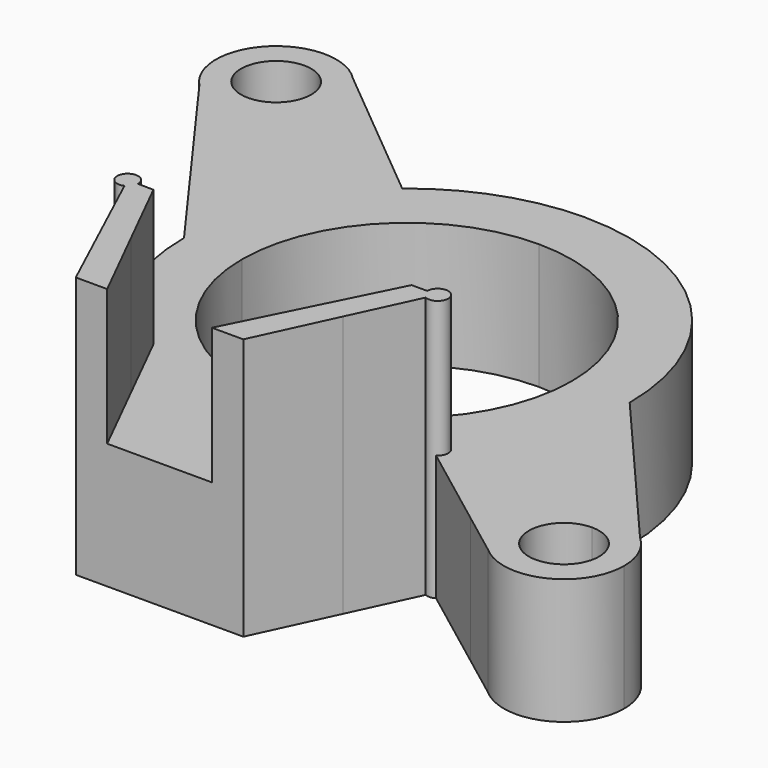
from build123d import *

# Parameters (mm, degrees)
F1_DEPTH = 12
F2_DEPTH = 25


with BuildPart() as f1:
    # F0 (on Top) → F1 (new body)
    with BuildSketch(Plane.XY):
        with BuildLine():
            ThreePointArc((-53.4150354704, 41.5196209399), (-52.7133447938, 40.4447331982), (-52.4674114412, 39.1848640586))
            Line((-52.4674114412, 39.1848640586), (-50.0674114412, 39.1848640586))
            ThreePointArc((-50.0674114412, 39.1848640586), (-50.4895358525, 41.3473260146), (-51.6939302973, 43.1922825863))
            Line((-51.6939302973, 43.1922825863), (-53.4150354704, 41.5196209399))
        make_face()
        with BuildLine():
            Line((-50.0674114412, 39.1848640586), (-52.4674114412, 39.1848640586))
            ThreePointArc((-52.4674114412, 39.1848640586), (-53.4486037242, 36.8160563416), (-55.8174114412, 35.8348640586))
            Line((-55.8174114412, 35.8348640586), (-55.8174114412, 33.4348640586))
            ThreePointArc((-55.8174114412, 33.4348640586), (-51.7515474493, 35.1190000668), (-50.0674114412, 39.1848640586))
        make_face()
        with BuildLine():
            ThreePointArc((-51.6939302973, 43.1922825863), (-50.4895358525, 41.3473260146), (-50.0674114412, 39.1848640586))
            Line((-50.0674114412, 39.1848640586), (-46.8600699283, 39.1848640586))
            Line((-46.8600699283, 39.1848640586), (-51.6939302973, 43.1922825863))
        make_face()
        with BuildLine():
            Line((-46.8600699283, 39.1848640586), (-50.0674114412, 39.1848640586))
            ThreePointArc((-50.0674114412, 39.1848640586), (-51.7515474493, 35.1190000668), (-55.8174114412, 33.4348640586))
            Line((-55.8174114412, 33.4348640586), (-55.8174114412, 29.501699648))
            Line((-55.8174114412, 29.501699648), (-45.4160998232, 15.1848640586))
            ThreePointArc((-45.4160998232, 15.1848640586), (-43.3893572478, 24.2490610317), (-37.6951490668, 31.5868635246))
            Line((-37.6951490668, 31.5868635246), (-46.8600699283, 39.1848640586))
        make_face()
        with BuildLine():
            Line((-55.8174114412, 33.4348640586), (-55.8174114412, 35.8348640586))
            ThreePointArc((-55.8174114412, 35.8348640586), (-57.1214560047, 36.099095471), (-58.219787412, 36.8501071773))
            Line((-58.219787412, 36.8501071773), (-59.9408925851, 35.177445531))
            ThreePointArc((-59.9408925851, 35.177445531), (-58.0556968861, 33.8883955874), (-55.8174114412, 33.4348640586))
        make_face()
        with BuildLine():
            ThreePointArc((-58.219787412, 36.8501071773), (-58.1521683225, 41.5872400294), (-53.4150354704, 41.5196209399))
            Line((-53.4150354704, 41.5196209399), (-51.6939302973, 43.1922825863))
            ThreePointArc((-51.6939302973, 43.1922825863), (-59.8248299688, 43.3083452025), (-59.9408925851, 35.177445531))
            Line((-59.9408925851, 35.177445531), (-58.219787412, 36.8501071773))
        make_face()
        with BuildLine():
            Line((-55.8174114412, 29.501699648), (-55.8174114412, 33.4348640586))
            ThreePointArc((-55.8174114412, 33.4348640586), (-58.0556968861, 33.8883955874), (-59.9408925851, 35.177445531))
            Line((-59.9408925851, 35.177445531), (-55.8174114412, 29.501699648))
        make_face()
        with BuildLine():
            ThreePointArc((-24.1338330771, 36.4671308048), (-31.3401896478, 35.2099309207), (-37.6951490668, 31.5868635246))
            ThreePointArc((-37.6951490668, 31.5868635246), (-43.3893572478, 24.2490610317), (-45.4160998232, 15.1848640586))
            Line((-45.4160998232, 15.1848640586), (-42.6338443592, 15.1848640586))
            Line((-42.6338443592, 15.1848640586), (-39.8838330771, 15.1848640586))
            ThreePointArc((-39.8838330771, 15.1848640586), (-35.2707648808, 26.3217958623), (-24.1338330771, 30.9348640586))
            Line((-24.1338330771, 30.9348640586), (-24.1338330771, 36.4671308048))
        make_face()
        with BuildLine():
            ThreePointArc((-2.8515663309, 15.1848640586), (-9.0849979418, 30.2336991939), (-24.1338330771, 36.4671308048))
            Line((-24.1338330771, 36.4671308048), (-24.1338330771, 30.9348640586))
            ThreePointArc((-24.1338330771, 30.9348640586), (-12.9969012734, 26.3217958623), (-8.3838330771, 15.1848640586))
            Line((-8.3838330771, 15.1848640586), (-5.6338443592, 15.1848640586))
            Line((-5.6338443592, 15.1848640586), (-2.8515663309, 15.1848640586))
        make_face()
        with BuildLine():
            Line((-42.6338443592, 15.1848640586), (-45.4160998232, 15.1848640586))
            ThreePointArc((-45.4160998232, 15.1848640586), (-43.9768109648, 7.4912884008), (-39.8536184288, 0.8383234878))
            ThreePointArc((-39.8536184288, 0.8383234878), (-38.7294279835, 1.3640933992), (-37.9593089049, 0.3908746355))
            ThreePointArc((-37.9593089049, 0.3908746355), (-37.9593613235, 0.3806357667), (-37.9595185738, 0.3703979712))
            Line((-37.9595185738, 0.3703979712), (-36.4598330771, 0.3396829748))
            Line((-36.4598330771, 0.3396829748), (-42.6338443592, 15.1848640586))
        make_face()
        with BuildLine():
            Line((7.549745287, 3.085096959), (-2.8515663309, 15.1848640586))
            Line((-2.8515663309, 15.1848640586), (-5.6338443592, 15.1848640586))
            Line((-5.6338443592, 15.1848640586), (-11.8078330771, 0.3396829748))
            Line((-11.8078330771, 0.3396829748), (-10.3078330771, 0.3396829748))
            ThreePointArc((-10.3078330771, 0.3396829748), (-9.3078330771, 1.3396829748), (-8.3078330771, 0.3396829748))
            ThreePointArc((-8.3078330771, 0.3396829748), (-8.4354300981, -0.1491043433), (-8.7856591617, -0.5131560499))
            Line((-8.7856591617, -0.5131560499), (-0.4328217774, -6.8151040581))
            Line((-0.4328217774, -6.8151040581), (1.9170580195, -6.8151040581))
            ThreePointArc((1.9170580195, -6.8151040581), (3.0940181915, -2.0251192122), (7.549745287, 0.0904625331))
            Line((7.549745287, 0.0904625331), (7.549745287, 3.085096959))
        make_face()
        with BuildLine():
            Line((-39.8838330771, 15.1848640586), (-42.6338443592, 15.1848640586))
            Line((-42.6338443592, 15.1848640586), (-36.4598330771, 0.3396829748))
            Line((-36.4598330771, 0.3396829748), (-29.3953061207, 0.3396829748))
            ThreePointArc((-29.3953061207, 0.3396829748), (-36.9971666349, 6.0965666504), (-39.8838330771, 15.1848640586))
        make_face()
        with BuildLine():
            ThreePointArc((-37.9593089049, 0.3908746355), (-38.7294279835, 1.3640933992), (-39.8536184288, 0.8383234878))
            ThreePointArc((-39.8536184288, 0.8383234878), (-39.649771274, 0.6181025887), (-39.4428392954, 0.4007778014))
            Line((-39.4428392954, 0.4007778014), (-38.9593089049, 0.3908746355))
            Line((-38.9593089049, 0.3908746355), (-37.9595185738, 0.3703979712))
            ThreePointArc((-37.9595185738, 0.3703979712), (-37.9593613235, 0.3806357667), (-37.9593089049, 0.3908746355))
        make_face()
        with BuildLine():
            ThreePointArc((-39.4428392954, 0.4007778014), (-39.649771274, 0.6181025887), (-39.8536184288, 0.8383234878))
            ThreePointArc((-39.8536184288, 0.8383234878), (-39.6769215407, -0.3055678279), (-38.5388324508, -0.5164288151))
            Line((-38.5388324508, -0.5164288151), (-38.5671831653, -0.4552536867))
            ThreePointArc((-38.5671831653, -0.4552536867), (-39.0111694362, -0.0335373263), (-39.4428392954, 0.4007778014))
        make_face()
        with BuildLine():
            Line((-5.6338443592, 15.1848640586), (-8.3838330771, 15.1848640586))
            ThreePointArc((-8.3838330771, 15.1848640586), (-11.2704995193, 6.0965666504), (-18.8723600334, 0.3396829748))
            Line((-18.8723600334, 0.3396829748), (-11.8078330771, 0.3396829748))
            Line((-11.8078330771, 0.3396829748), (-5.6338443592, 15.1848640586))
        make_face()
        with BuildLine():
            Line((11.3814063915, -1.3722454101), (7.549745287, 3.085096959))
            Line((7.549745287, 3.085096959), (7.549745287, 0.0904625331))
            ThreePointArc((7.549745287, 0.0904625331), (9.6004245249, -0.2876463043), (11.3814063915, -1.3722454101))
        make_face()
        with BuildLine():
            Line((-29.3953061207, 0.3396829748), (-36.4598330771, 0.3396829748))
            Line((-36.4598330771, 0.3396829748), (-32.8884867815, -6.8151040581))
            Line((-32.8884867815, -6.8151040581), (-24.1338330771, -6.8151040581))
            Line((-24.1338330771, -6.8151040581), (-24.1338330771, -0.5651359414))
            ThreePointArc((-24.1338330771, -0.5651359414), (-26.8031867376, -0.3372830556), (-29.3953061207, 0.3396829748))
        make_face()
        with BuildLine():
            Line((-32.8884867815, -6.8151040581), (-36.4598330771, 0.3396829748))
            Line((-36.4598330771, 0.3396829748), (-37.9595185738, 0.3703979712))
            ThreePointArc((-37.9595185738, 0.3703979712), (-38.1221082882, -0.1560212663), (-38.5388324508, -0.5164288151))
            Line((-38.5388324508, -0.5164288151), (-35.6198039494, -6.8151040581))
            Line((-35.6198039494, -6.8151040581), (-32.8884867815, -6.8151040581))
        make_face()
        with BuildLine():
            Line((-38.9593089049, 0.3908746355), (-39.4428392954, 0.4007778014))
            ThreePointArc((-39.4428392954, 0.4007778014), (-39.0111694362, -0.0335373263), (-38.5671831653, -0.4552536867))
            Line((-38.5671831653, -0.4552536867), (-38.9593089049, 0.3908746355))
        make_face()
        with BuildLine():
            Line((-38.5671831653, -0.4552536867), (-38.5388324508, -0.5164288151))
            ThreePointArc((-38.5388324508, -0.5164288151), (-38.1221082882, -0.1560212663), (-37.9595185738, 0.3703979712))
            Line((-37.9595185738, 0.3703979712), (-38.9593089049, 0.3908746355))
            Line((-38.9593089049, 0.3908746355), (-38.5671831653, -0.4552536867))
        make_face()
        with BuildLine():
            Line((-11.8078330771, 0.3396829748), (-18.8723600334, 0.3396829748))
            ThreePointArc((-18.8723600334, 0.3396829748), (-21.4644794165, -0.3372830556), (-24.1338330771, -0.5651359414))
            Line((-24.1338330771, -0.5651359414), (-24.1338330771, -6.8151040581))
            Line((-24.1338330771, -6.8151040581), (-15.3791793726, -6.8151040581))
            Line((-15.3791793726, -6.8151040581), (-11.8078330771, 0.3396829748))
        make_face()
        with BuildLine():
            Line((-10.3078330771, 0.3396829748), (-11.8078330771, 0.3396829748))
            Line((-11.8078330771, 0.3396829748), (-15.3791793726, -6.8151040581))
            Line((-15.3791793726, -6.8151040581), (-12.6354347442, -6.8151040581))
            Line((-12.6354347442, -6.8151040581), (-9.7295423368, -0.5670481321))
            ThreePointArc((-9.7295423368, -0.5670481321), (-10.1509550314, -0.1980394165), (-10.3078330771, 0.3396829748))
        make_face()
        with BuildLine():
            ThreePointArc((11.3814063915, -1.3722454101), (9.6004245249, -0.2876463043), (7.549745287, 0.0904625331))
            Line((7.549745287, 0.0904625331), (7.549745287, -2.3095374669))
            ThreePointArc((7.549745287, -2.3095374669), (8.744488843, -2.5298269634), (9.7821043653, -3.1617238338))
            Line((9.7821043653, -3.1617238338), (11.3814063915, -1.3722454101))
        make_face()
        with BuildLine():
            Line((7.549745287, -2.3095374669), (7.549745287, 0.0904625331))
            ThreePointArc((7.549745287, 0.0904625331), (3.0940181915, -2.0251192122), (1.9170580195, -6.8151040581))
            ThreePointArc((1.9170580195, -6.8151040581), (2.5652294004, -8.526086154), (3.7180841826, -9.9468295237))
            Line((3.7180841826, -9.9468295237), (5.3173862088, -8.1573511))
            ThreePointArc((5.3173862088, -8.1573511), (4.4200347836, -4.4647939109), (7.549745287, -2.3095374669))
        make_face()
        with BuildLine():
            ThreePointArc((13.299745287, -5.6595374669), (12.7982951511, -3.3110859931), (11.3814063915, -1.3722454101))
            Line((11.3814063915, -1.3722454101), (9.7821043653, -3.1617238338))
            ThreePointArc((9.7821043653, -3.1617238338), (10.6075960774, -4.291309217), (10.899745287, -5.6595374669))
            ThreePointArc((10.899745287, -5.6595374669), (8.917973537, -8.7173882573), (5.3173862088, -8.1573511))
            Line((5.3173862088, -8.1573511), (3.7180841826, -9.9468295237))
            ThreePointArc((3.7180841826, -9.9468295237), (9.8981967608, -10.9080873309), (13.299745287, -5.6595374669))
        make_face()
        Polygon((-24.1338330771, -6.8151040581), (-32.8884867815, -6.8151040581), (-29.1338330771, -14.3371266833), (-24.1338330771, -14.3371266833), (-24.1338330771, -7.8529477167), align=None)
        Polygon((-29.1338330771, -14.3371266833), (-32.8884867815, -6.8151040581), (-35.6198039494, -6.8151040581), (-32.1338330771, -14.3371266833), align=None)
        Polygon((-12.6354347442, -6.8151040581), (-15.3791793726, -6.8151040581), (-19.1338330771, -14.3371266833), (-16.1338330771, -14.3371266833), align=None)
        Polygon((-19.1338330771, -14.3371266833), (-15.3791793726, -6.8151040581), (-24.1338330771, -6.8151040581), (-24.1338330771, -7.8529477167), (-24.1338330771, -14.3371266833), align=None)
        with BuildLine():
            ThreePointArc((-8.3078330771, 0.3396829748), (-9.3078330771, 1.3396829748), (-10.3078330771, 0.3396829748))
            Line((-10.3078330771, 0.3396829748), (-9.3078330771, 0.3396829748))
            Line((-9.3078330771, 0.3396829748), (-9.4658153661, 0))
            Line((-9.4658153661, 0), (-8.7856591617, -0.5131560499))
            ThreePointArc((-8.7856591617, -0.5131560499), (-8.4354300981, -0.1491043433), (-8.3078330771, 0.3396829748))
        make_face()
        with BuildLine():
            Line((-9.3078330771, 0.3396829748), (-10.3078330771, 0.3396829748))
            ThreePointArc((-10.3078330771, 0.3396829748), (-10.1509550314, -0.1980394165), (-9.7295423368, -0.5670481321))
            Line((-9.7295423368, -0.5670481321), (-9.4658153661, 0))
            Line((-9.4658153661, 0), (-9.3078330771, 0.3396829748))
        make_face()
        with BuildLine():
            ThreePointArc((3.7180841826, -9.9468295237), (2.5652294004, -8.526086154), (1.9170580195, -6.8151040581))
            Line((1.9170580195, -6.8151040581), (-0.4328217774, -6.8151040581))
            Line((-0.4328217774, -6.8151040581), (3.7180841826, -9.9468295237))
        make_face()
        with BuildLine():
            Line((-9.4658153661, 0), (-9.7295423368, -0.5670481321))
            ThreePointArc((-9.7295423368, -0.5670481321), (-9.2508297799, -0.6586910153), (-8.7856591617, -0.5131560499))
            Line((-8.7856591617, -0.5131560499), (-9.4658153661, 0))
        make_face()
    extrude(amount=F1_DEPTH)

    # F0 (on Top) → F2 (join)
    with BuildSketch(Plane.XY):
        Polygon((-29.1338330771, -14.3371266833), (-32.8884867815, -6.8151040581), (-35.6198039494, -6.8151040581), (-32.1338330771, -14.3371266833), align=None)
        with BuildLine():
            Line((-32.8884867815, -6.8151040581), (-36.4598330771, 0.3396829748))
            Line((-36.4598330771, 0.3396829748), (-37.9595185738, 0.3703979712))
            ThreePointArc((-37.9595185738, 0.3703979712), (-38.1221082882, -0.1560212663), (-38.5388324508, -0.5164288151))
            Line((-38.5388324508, -0.5164288151), (-35.6198039494, -6.8151040581))
            Line((-35.6198039494, -6.8151040581), (-32.8884867815, -6.8151040581))
        make_face()
        with BuildLine():
            Line((-38.5671831653, -0.4552536867), (-38.5388324508, -0.5164288151))
            ThreePointArc((-38.5388324508, -0.5164288151), (-38.1221082882, -0.1560212663), (-37.9595185738, 0.3703979712))
            Line((-37.9595185738, 0.3703979712), (-38.9593089049, 0.3908746355))
            Line((-38.9593089049, 0.3908746355), (-38.5671831653, -0.4552536867))
        make_face()
        with BuildLine():
            ThreePointArc((-37.9593089049, 0.3908746355), (-38.7294279835, 1.3640933992), (-39.8536184288, 0.8383234878))
            ThreePointArc((-39.8536184288, 0.8383234878), (-39.649771274, 0.6181025887), (-39.4428392954, 0.4007778014))
            Line((-39.4428392954, 0.4007778014), (-38.9593089049, 0.3908746355))
            Line((-38.9593089049, 0.3908746355), (-37.9595185738, 0.3703979712))
            ThreePointArc((-37.9595185738, 0.3703979712), (-37.9593613235, 0.3806357667), (-37.9593089049, 0.3908746355))
        make_face()
        with BuildLine():
            ThreePointArc((-39.4428392954, 0.4007778014), (-39.649771274, 0.6181025887), (-39.8536184288, 0.8383234878))
            ThreePointArc((-39.8536184288, 0.8383234878), (-39.6769215407, -0.3055678279), (-38.5388324508, -0.5164288151))
            Line((-38.5388324508, -0.5164288151), (-38.5671831653, -0.4552536867))
            ThreePointArc((-38.5671831653, -0.4552536867), (-39.0111694362, -0.0335373263), (-39.4428392954, 0.4007778014))
        make_face()
        with BuildLine():
            Line((-38.9593089049, 0.3908746355), (-39.4428392954, 0.4007778014))
            ThreePointArc((-39.4428392954, 0.4007778014), (-39.0111694362, -0.0335373263), (-38.5671831653, -0.4552536867))
            Line((-38.5671831653, -0.4552536867), (-38.9593089049, 0.3908746355))
        make_face()
        with BuildLine():
            Line((-9.3078330771, 0.3396829748), (-10.3078330771, 0.3396829748))
            ThreePointArc((-10.3078330771, 0.3396829748), (-10.1509550314, -0.1980394165), (-9.7295423368, -0.5670481321))
            Line((-9.7295423368, -0.5670481321), (-9.4658153661, 0))
            Line((-9.4658153661, 0), (-9.3078330771, 0.3396829748))
        make_face()
        with BuildLine():
            ThreePointArc((-8.3078330771, 0.3396829748), (-9.3078330771, 1.3396829748), (-10.3078330771, 0.3396829748))
            Line((-10.3078330771, 0.3396829748), (-9.3078330771, 0.3396829748))
            Line((-9.3078330771, 0.3396829748), (-9.4658153661, 0))
            Line((-9.4658153661, 0), (-8.7856591617, -0.5131560499))
            ThreePointArc((-8.7856591617, -0.5131560499), (-8.4354300981, -0.1491043433), (-8.3078330771, 0.3396829748))
        make_face()
        with BuildLine():
            Line((-9.4658153661, 0), (-9.7295423368, -0.5670481321))
            ThreePointArc((-9.7295423368, -0.5670481321), (-9.2508297799, -0.6586910153), (-8.7856591617, -0.5131560499))
            Line((-8.7856591617, -0.5131560499), (-9.4658153661, 0))
        make_face()
        with BuildLine():
            Line((-10.3078330771, 0.3396829748), (-11.8078330771, 0.3396829748))
            Line((-11.8078330771, 0.3396829748), (-15.3791793726, -6.8151040581))
            Line((-15.3791793726, -6.8151040581), (-12.6354347442, -6.8151040581))
            Line((-12.6354347442, -6.8151040581), (-9.7295423368, -0.5670481321))
            ThreePointArc((-9.7295423368, -0.5670481321), (-10.1509550314, -0.1980394165), (-10.3078330771, 0.3396829748))
        make_face()
        Polygon((-12.6354347442, -6.8151040581), (-15.3791793726, -6.8151040581), (-19.1338330771, -14.3371266833), (-16.1338330771, -14.3371266833), align=None)
    extrude(amount=F2_DEPTH)


solid = f1.part
